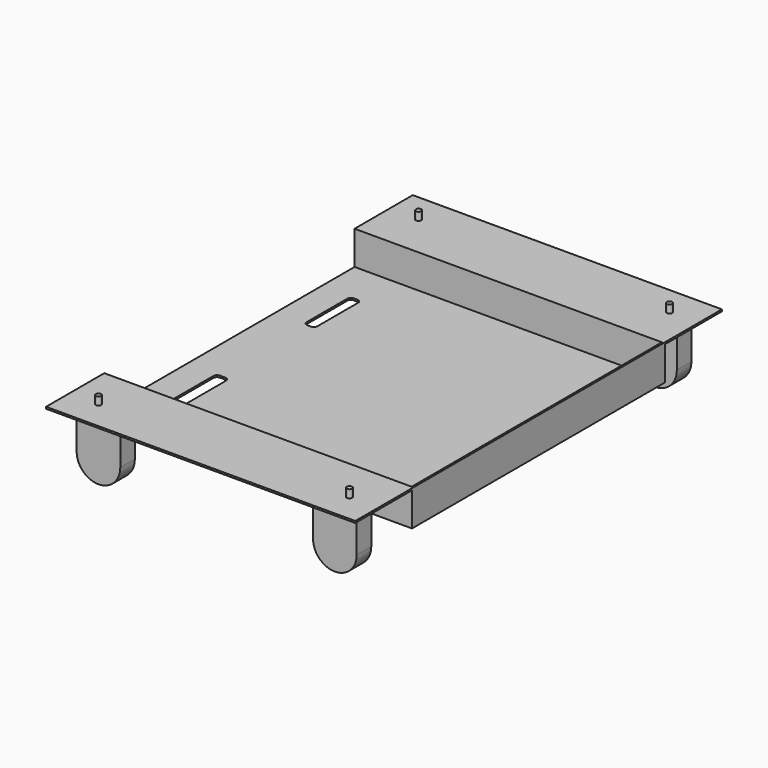
from build123d import *

# Parameters (mm, degrees)
F0_W      = 539.75
F0_H      = 552.45
F1_DEPTH  = 3.175
F3_DEPTH  = 58.7375
F4_W      = 539.75
F4_H      = 127
F4_R      = 4.7625
F5_DEPTH  = 3.175
F6_R      = 4.699
F7_DEPTH  = 17.145
F8_R      = 25.4
F9_DEPTH  = 1.651
F10_W     = 76.2
F10_H     = 31.75
F11_DEPTH = 107.8865
F12_R     = 38.09999
F13_W     = 3.175
F13_H     = 546.1
F14_DEPTH = 31.75


# Not quite as in the source:
# - a fillet or chamfer is up to 0.001 mm smaller than in the source, because OpenCascade refuses the exact size


with BuildPart() as f1:
    # F0 (on Top) → F1 (new body)
    with BuildSketch(Plane.XY):
        Rectangle(F0_W, F0_H)
        with BuildLine():
            ThreePointArc((-219.075, -98.425), (-217.2151280605, -93.9348719395), (-212.725, -92.075))
            Line((-212.725, -92.075), (-203.2, -92.075))
            ThreePointArc((-203.2, -92.075), (-198.7098719395, -93.9348719395), (-196.85, -98.425))
            Line((-196.85, -98.425), (-196.85, -193.675))
            ThreePointArc((-196.85, -193.675), (-198.7098719395, -198.1651280605), (-203.2, -200.025))
            Line((-203.2, -200.025), (-212.725, -200.025))
            ThreePointArc((-212.725, -200.025), (-217.2151280605, -198.1651280605), (-219.075, -193.675))
            Line((-219.075, -193.675), (-219.075, -98.425))
        make_face(mode=Mode.SUBTRACT)
        with BuildLine():
            ThreePointArc((-219.075, 193.675), (-217.2151280605, 198.1651280605), (-212.725, 200.025))
            Line((-212.725, 200.025), (-206.375, 200.025))
            ThreePointArc((-206.375, 200.025), (-201.8848719395, 198.1651280605), (-200.025, 193.675))
            Line((-200.025, 193.675), (-200.025, 104.775))
            ThreePointArc((-200.025, 104.775), (-201.8848719395, 100.2848719395), (-206.375, 98.425))
            Line((-206.375, 98.425), (-212.725, 98.425))
            ThreePointArc((-212.725, 98.425), (-217.2151280605, 100.2848719395), (-219.075, 104.775))
            Line((-219.075, 104.775), (-219.075, 193.675))
        make_face(mode=Mode.SUBTRACT)
    extrude(amount=F1_DEPTH)

    # F2 (on face) → F3 (join)
    with BuildSketch(Plane.XY.offset(3.175)):
        Polygon((-269.875, 276.225), (-269.875, 273.05), (266.7, 273.05), (266.7, -273.05), (-269.875, -273.05), (-269.875, -276.225), (269.875, -276.225), (269.875, 276.225), align=None)
    extrude(amount=F3_DEPTH)

    # F4 (on face) → F5 (join)
    with BuildSketch(Plane.XY.offset(61.9125)):
        with Locations((0, 336.55)):
            Rectangle(F4_W, F4_H)
        with Locations((-219.075, 349.25)):
            Circle(F4_R, mode=Mode.SUBTRACT)
        with Locations((219.075, 349.25)):
            Circle(F4_R, mode=Mode.SUBTRACT)
        with Locations((0, -336.55)):
            Rectangle(F4_W, F4_H)
        with Locations((-219.075, -349.25)):
            Circle(F4_R, mode=Mode.SUBTRACT)
        with Locations((219.075, -349.25)):
            Circle(F4_R, mode=Mode.SUBTRACT)
    extrude(amount=-F5_DEPTH)



with BuildPart() as f7:
    # F6 (on face) → F7 (new body)
    with BuildSketch(Plane(origin=(0, 0, 58.7375), x_dir=(1, 0, 0), z_dir=(0, 0, -1))):
        with Locations((-219.075, 349.25)):
            Circle(F6_R)
    extrude(amount=-F7_DEPTH)


with BuildPart() as f7b:
    # F6 (on face) → F7, piece 2 (new body)
    with BuildSketch(Plane(origin=(0, 0, 58.7375), x_dir=(1, 0, 0), z_dir=(0, 0, -1))):
        with Locations((219.075, 349.25)):
            Circle(F6_R)
    extrude(amount=-F7_DEPTH)


with BuildPart() as f7c:
    # F6 (on face) → F7, piece 3 (new body)
    with BuildSketch(Plane(origin=(0, 0, 58.7375), x_dir=(1, 0, 0), z_dir=(0, 0, -1))):
        with Locations((-219.075, -349.25)):
            Circle(F6_R)
    extrude(amount=-F7_DEPTH)


with BuildPart() as f7d:
    # F6 (on face) → F7, piece 4 (new body)
    with BuildSketch(Plane(origin=(0, 0, 58.7375), x_dir=(1, 0, 0), z_dir=(0, 0, -1))):
        with Locations((219.075, -349.25)):
            Circle(F6_R)
    extrude(amount=-F7_DEPTH)


with BuildPart() as f1_1:
    add(f1.part)

    add(f7.part)  # F9 merges F7

    add(f7b.part)  # F9 merges F7b

    add(f7c.part)  # F9 merges F7c

    add(f7d.part)  # F9 merges F7d
    # F8 (on face) → F9 (join)
    with BuildSketch(Plane(origin=(0, 0, 58.7375), x_dir=(1, 0, 0), z_dir=(0, 0, -1))):
        with Locations((-219.075, 349.25)):
            Circle(F8_R)
        with Locations((219.075, 349.25)):
            Circle(F8_R)
        with Locations((-219.075, -349.25)):
            Circle(F8_R)
        with Locations((219.075, -349.25)):
            Circle(F8_R)
    extrude(amount=F9_DEPTH)

    # F10 (on face) → F11 (join)
    with BuildSketch(Plane(origin=(0, 0, 57.0865), x_dir=(1, 0, 0), z_dir=(0, 0, -1))):
        with Locations((-206.375, 349.25)):
            Rectangle(F10_W, F10_H)
        with Locations((206.375, 349.25)):
            Rectangle(F10_W, F10_H)
        with Locations((-206.375, -349.25)):
            Rectangle(F10_W, F10_H)
        with Locations((206.375, -349.25)):
            Rectangle(F10_W, F10_H)
    extrude(amount=F11_DEPTH)

    # F12 (radius 38.1 in the source; OpenCascade refuses exactly that, so slightly less here)
    f12_edges = [f1_1.edges().sort_by_distance(p)[0] for p in [
        (-168.275, -349.25, -50.8),
        (-244.475, -349.25, -50.8),
        (168.275, -349.25, -50.8),
        (244.475, -349.25, -50.8),
        (-244.475, 349.25, -50.8),
        (-168.275, 349.25, -50.8),
        (168.275, 349.25, -50.8),
        (244.475, 349.25, -50.8),
    ]]
    fillet(f12_edges, radius=F12_R)

    # F13 (on face) → F14 (join)
    with BuildSketch(Plane.XY.offset(3.175)):
        with Locations((-268.2875, 0)):
            Rectangle(F13_W, F13_H)
    extrude(amount=-F14_DEPTH)


solid = f1_1.part
